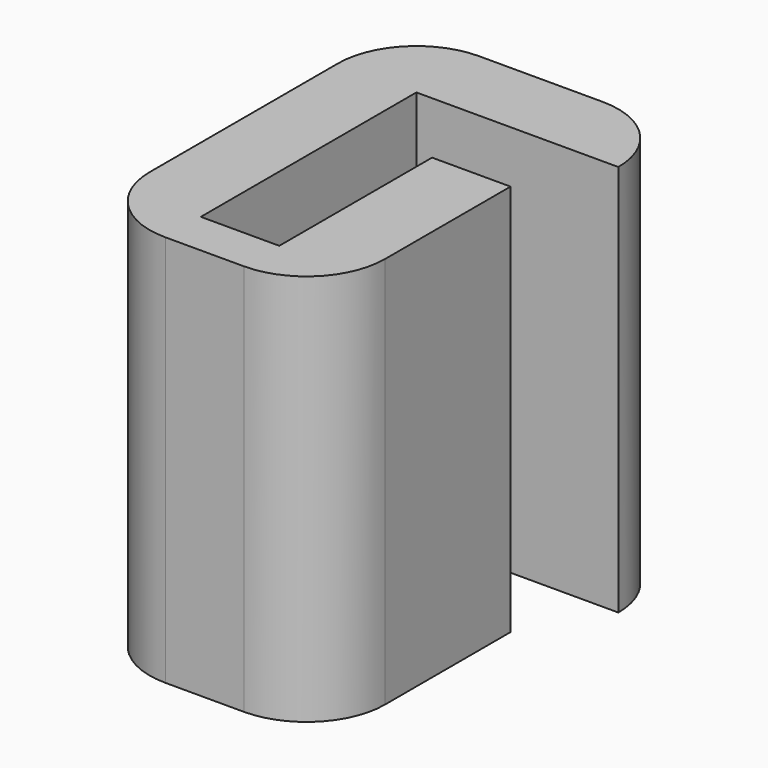
from build123d import *

# Parameters (mm, degrees)
F0_W     = 5
F0_H     = 5
F0_W_2   = 12.8715214133
F0_H_2   = 2.8254000843
F1_DEPTH = 25
F2_R     = 4.99999


# Not quite as in the source:
# - a fillet or chamfer is up to 0.001 mm smaller than in the source, because OpenCascade refuses the exact size


with BuildPart() as f1:
    # F0 (on Top) → F1 (new body)
    with BuildSketch(Plane.XY):
        with Locations((2.5, -2.5)):
            Rectangle(F0_W, F0_H)
        with Locations((11.4357607067, -2.5)):
            Rectangle(F0_W_2, F0_H)
        Polygon((5, -5), (0, -5), (0, -25), (5, -25), (5, -22.1745999157), align=None)
        with Locations((7.5, -23.5872999579)):
            Rectangle(F0_W, F0_H_2)
        Polygon((10, -10), (10, -22.1745999157), (10, -25), (15, -25), (15, -10), align=None)
    extrude(amount=F1_DEPTH)

    # F2 (radius 5 in the source; OpenCascade refuses exactly that, so slightly less here)
    f2_edges = [f1.edges().sort_by_distance(p)[0] for p in [
        (0, 0, 12.5),
        (0, -25, 12.5),
        (15, -25, 12.5),
        (17.871521, 0, 12.5),
    ]]
    fillet(f2_edges, radius=F2_R)


solid = f1.part
